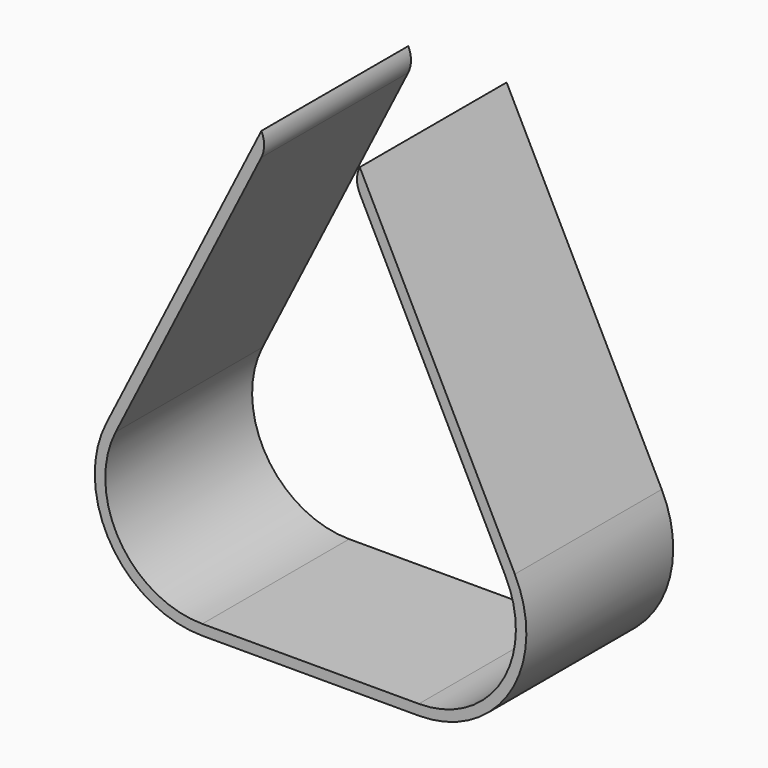
from build123d import *

# Parameters (mm, degrees)
F1_DEPTH    = 35
F2_T1_DEPTH = 55


# Not quite as in the source:
# - a fillet or chamfer that OpenCascade refuses, or shapes differently, is made with other operations: its cross-section is extruded or revolved along the edge and cut away or added


with BuildPart() as f1:
    # F0 (on Front) → F1 (new body)
    with BuildSketch(Plane.XZ):
        with BuildLine():
            Line((-15.5290191181, 81.5544475097), (-17.315076228, 80.6544475097))
            Line((-17.315076228, 80.6544475097), (12.2598850951, 21.9627031234))
            ThreePointArc((12.2598850951, 21.9627031234), (11.4910392166, 3.9362212778), (-4.2611431719, -4.8622968766))
            Line((-4.2611431719, -4.8622968766), (-45.5504947187, -4.8622968766))
            ThreePointArc((-45.5504947187, -4.8622968766), (-61.3026771072, 3.9362212778), (-62.0715229858, 21.9627031234))
            Line((-62.0715229858, 21.9627031234), (-32.4965616626, 80.6544475097))
            Line((-32.4965616626, 80.6544475097), (-34.2826187726, 81.5544475097))
            Line((-34.2826187726, 81.5544475097), (-63.8575800957, 22.8627031234))
            ThreePointArc((-63.8575800957, 22.8627031234), (-63.0056157438, 2.8874124296), (-45.5504947187, -6.8622968766))
            Line((-45.5504947187, -6.8622968766), (-4.2611431719, -6.8622968766))
            ThreePointArc((-4.2611431719, -6.8622968766), (13.1939778532, 2.8874124296), (14.0459422051, 22.8627031234))
            Line((14.0459422051, 22.8627031234), (-15.5290191181, 81.5544475097))
        make_face()
    extrude(amount=F1_DEPTH)

    # F2: fillet of radius 5 on 2 edges, made by hand

    # F2_s2 → F2_t1 (cut)
    with BuildSketch(Plane.XZ.offset(-10)):
        with BuildLine():
            ThreePointArc((-34.2965616626, 77.0823332898), (-33.7617287381, 79.3167446648), (-34.2826187726, 81.5544475097))
            Line((-34.2826187726, 81.5544475097), (-32.4965616626, 80.6544475097))
            Line((-32.4965616626, 80.6544475097), (-34.2965616626, 77.0823332898))
        make_face()
        with BuildLine():
            ThreePointArc((-15.5290191181, 81.5544475097), (-16.0499091526, 79.3167446648), (-15.515076228, 77.0823332898))
            Line((-15.515076228, 77.0823332898), (-17.315076228, 80.6544475097))
            Line((-17.315076228, 80.6544475097), (-15.5290191181, 81.5544475097))
        make_face()
    extrude(amount=F2_T1_DEPTH, mode=Mode.SUBTRACT)


solid = f1.part
